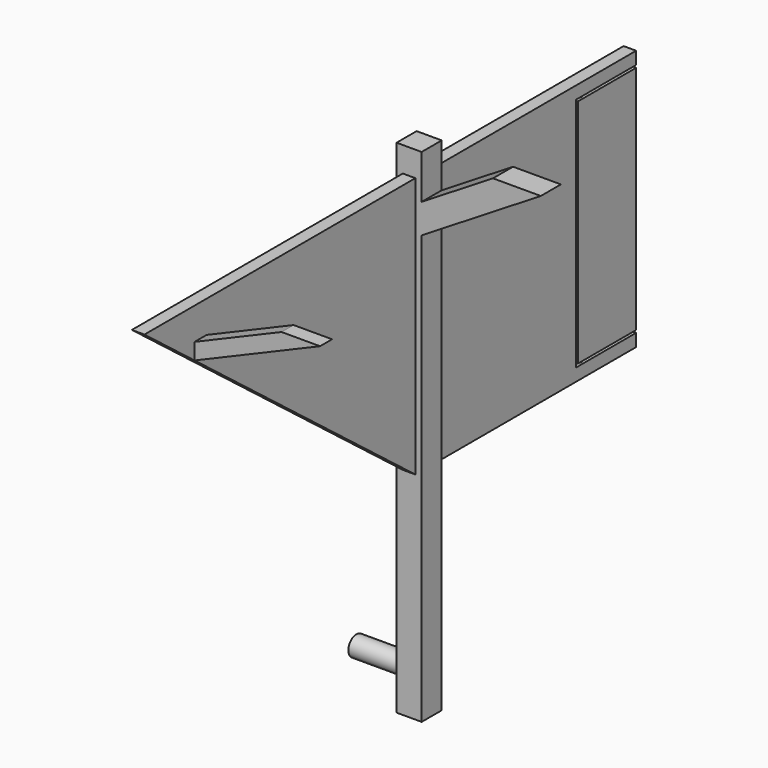
from build123d import *

# Parameters (mm, degrees)
F0_W      = 10
F0_H      = 200
F1_DEPTH  = 10
F3_DEPTH  = 135
F5_DEPTH  = 7.501
F6_W      = 5
F6_H      = 10
F6_H_2    = 9.253
F7_DEPTH  = 57.5
F9_DEPTH  = 30
F11_DEPTH = 100
F13_DEPTH = 5
F15_DEPTH = 92
F17_DEPTH = 94
F19_DEPTH = 25
F20_W     = 6
F20_H     = 6
F20_H_2   = 7.253
F20_H_3   = 2
F21_DEPTH = 50
F23_DEPTH = 25


# Not quite as in the source:
# - a feature names something its author has since deleted; it is built from what else it names


with BuildPart() as f1:
    # F0 (on Front) → F1 (new body)
    with BuildSketch(Plane.XZ):
        Rectangle(F0_W, F0_H)
    extrude(amount=F1_DEPTH)

    # F2 (on face) → F3 (join)
    with BuildSketch(Plane.XZ.offset(10)):
        Polygon((2.5, 90), (0, 90), (-2.5, 90), (-2.5, -14), (0, -14), (2.5, -14), align=None)
    extrude(amount=F3_DEPTH)

    # F4 (on face) → F5 (cut, through all)
    with BuildSketch(Plane.YZ.offset(2.5)):
        Polygon((-10, -14), (-145, 90), (-145, -14), align=None)
    extrude(amount=-F5_DEPTH, mode=Mode.SUBTRACT)

    # F6 (on face) → F7 (join)
    with BuildSketch(Plane(origin=(-5, 0, 0), x_dir=(0, -1, 0), z_dir=(-1, 0, 0))):
        with Locations((7.5, 75.747)):
            Rectangle(F6_W, F6_H)
        with Locations((2.5, 75.747)):
            Rectangle(F6_W, F6_H)
        with Locations((2.5, 85.3735)):
            Rectangle(F6_W, F6_H_2)
        with Locations((7.5, 85.3735)):
            Rectangle(F6_W, F6_H_2)
        with Locations((2.5, 95)):
            Rectangle(F6_W, F6_H)
        with Locations((7.5, 95)):
            Rectangle(F6_W, F6_H)
    extrude(amount=-F7_DEPTH)

    # F8 (on face) → F9 (join)
    with BuildSketch(Plane.YZ.offset(5)):
        with BuildLine():
            ThreePointArc((-1, -85), (-7.8284271247, -82.1715728753), (-5, -89))
            ThreePointArc((-5, -89), (-2.1715728753, -87.8284271247), (-1, -85))
        make_face()
    extrude(amount=-F9_DEPTH)

    # F10 (on face) → F11 (join)
    with BuildSketch(Plane(origin=(0, 0, 0), x_dir=(-1, 0, 0), z_dir=(0, 1, 0))):
        Polygon((2.5, 90), (0, 90), (-2.5, 90), (-2.5, -14), (2.5, -14), align=None)
    extrude(amount=F11_DEPTH)

    # F12 (on face) → F13 (cut, through all)
    with BuildSketch(Plane.YZ.offset(2.5)):
        Polygon((100, 84), (100, 85), (70, 85), (70, -9), (100, -9), (100, -8), (71, -8), (71, 84), align=None)
    extrude(amount=-F13_DEPTH, mode=Mode.SUBTRACT)

    # F14 (on face) → F15 (cut, through all)
    with BuildSketch(Plane.XY.offset(84)):
        with BuildLine():
            ThreePointArc((0, 72.5), (1.0606601718, 72.9393398282), (1.5, 74))
            ThreePointArc((1.5, 74), (-1.0606601718, 75.0606601718), (0, 72.5))
        make_face()
    extrude(amount=-F15_DEPTH, mode=Mode.SUBTRACT)

    # F18 (on face) → F19 (cut)
    with BuildSketch(Plane.XZ.offset(10)):
        Polygon((5, 100), (5, 82.4912516314), (33.4300942641, 100), align=None)
        Polygon((52.5, 100), (5, 70.747), (52.5, 70.747), align=None)
    extrude(amount=-F19_DEPTH, mode=Mode.SUBTRACT)

    # F20 (on face) → F21 (join)
    with BuildSketch(Plane.YZ.offset(2.5)):
        with Locations((-117, 73.747)):
            Rectangle(F20_W, F20_H)
        with Locations((-117, 80.3735)):
            Rectangle(F20_W, F20_H_2)
        with Locations((-117, 87)):
            Rectangle(F20_W, F20_H)
        with Locations((-117, 91)):
            Rectangle(F20_W, F20_H_3)
    extrude(amount=F21_DEPTH)

    # F22 (on face) → F23 (cut)
    with BuildSketch(Plane.XZ.offset(120)):
        Polygon((2.5, 90), (2.5, 77.2665349627), (37.1620830878, 92), (2.5, 92), align=None)
        Polygon((52.5, 92), (2.5, 70.747), (52.5, 70.747), align=None)
    extrude(amount=-F23_DEPTH, mode=Mode.SUBTRACT)


with BuildPart() as f17:
    # F16 (on face) → F17 (new body, through all)
    with BuildSketch(Plane(origin=(0, 0, 85), x_dir=(1, 0, 0), z_dir=(0, 0, -1))):
        with BuildLine():
            ThreePointArc((1.5, -74), (1.0606601718, -72.9393398282), (0, -72.5))
            Line((0, -72.5), (0, -74))
            Line((0, -74), (0, -75.5))
            ThreePointArc((0, -75.5), (1.0606601718, -75.0606601718), (1.5, -74))
        make_face()
        with BuildLine():
            Line((0, -74), (0, -72.5))
            ThreePointArc((0, -72.5), (-1.5, -74), (0, -75.5))
            Line((0, -75.5), (0, -74))
        make_face()
    extrude(amount=F17_DEPTH)


solid = Compound([f1.part, f17.part])
